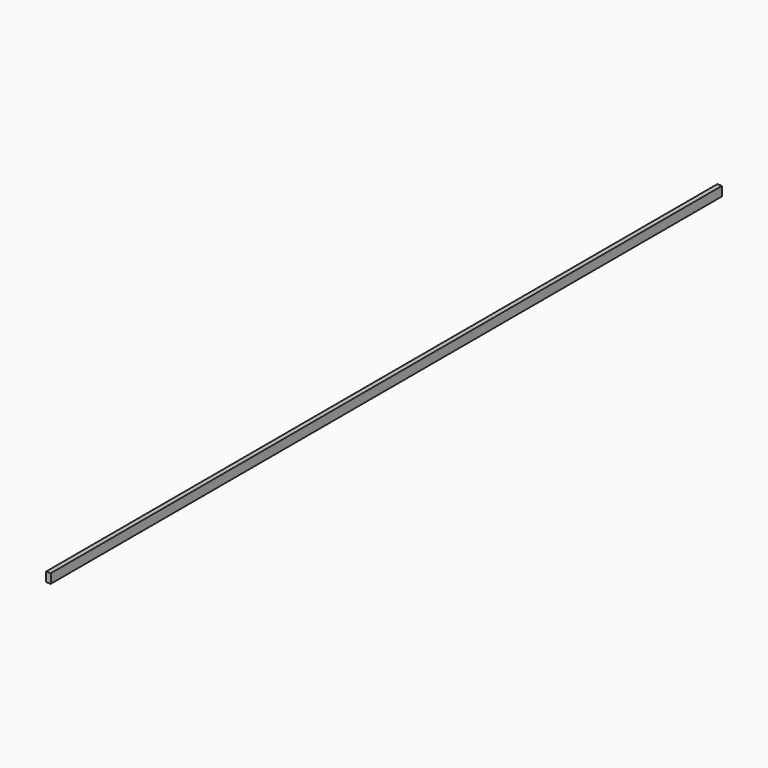
from build123d import *

# Parameters (mm, degrees)
F0_W     = 15.875
F0_H     = 31.75
F1_DEPTH = 2851.15


# Not quite as in the source:
# - a feature names something its author has since deleted; it is built from what else it names


with BuildPart() as f1:
    # F0 (on Front) → F1 (new body)
    with BuildSketch(Plane.XZ):
        with Locations((7.9375, -15.875)):
            Rectangle(F0_W, F0_H)
    extrude(amount=F1_DEPTH)


solid = f1.part
